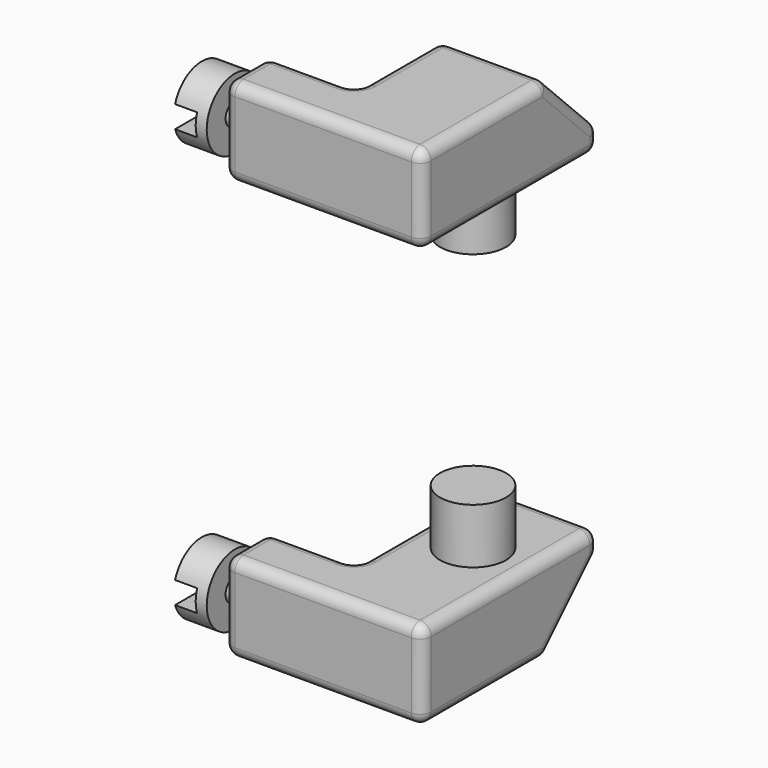
from build123d import *

# Parameters (mm, degrees)
F0_W      = 5
F0_H      = 10
F1_DEPTH  = 4
F2_SIZE   = 3
F3_R      = 1.5
F4_DEPTH  = 2.5
F5_W      = 2.5
F5_H      = 4
F6_DEPTH  = 4
F7_R      = 0.5
F8_R      = 0.5269864315
F9_DEPTH  = 0.5
F10_R     = 1.5960368508
F11_DEPTH = 1.5
F12_W     = 4.0138932984
F12_H     = 1
F13_DEPTH = 1


with BuildPart() as f1:
    # F0 (on Top) → F1 (new body)
    with BuildSketch(Plane.XY):
        Rectangle(F0_W, F0_H)
    extrude(amount=F1_DEPTH)

    # F2
    f2_edges = [f1.edges().sort_by_distance(p)[0] for p in [
        (0, 5, 4),
    ]]
    chamfer(f2_edges, length=F2_SIZE)

    # F3 (on face) → F4 (join)
    with BuildSketch(Plane(origin=(0, 0, 0), x_dir=(1, 0, 0), z_dir=(0, 0, -1))):
        with Locations((0, -1)):
            Circle(F3_R)
    extrude(amount=F4_DEPTH)

    # F5 (on face) → F6 (join)
    with BuildSketch(Plane(origin=(-2.5, 0, 0), x_dir=(0, -1, 0), z_dir=(-1, 0, 0))):
        with Locations((3.75, 2)):
            Rectangle(F5_W, F5_H)
    extrude(amount=F6_DEPTH)

    # F7
    f7_edges = [f1.edges().sort_by_distance(p)[0] for p in [
        (-2.5, -2.5, 2),
        (2.5, -5, 2),
        (0, 5, 0),
        (0, 5, 1),
        (2.5, 3.5, 2.5),
        (0, 2, 4),
        (2.5, 5, 0.5),
        (-2.5, 3.5, 2.5),
        (-2.5, 5, 0.5),
        (-2.5, 1.25, 0),
        (2.5, 0, 0),
        (-2, -5, 0),
        (-2, -5, 4),
        (2.5, -1.5, 4),
        (-2.5, -0.25, 4),
        (-6.5, -5, 2),
        (-6.5, -3.75, 4),
        (-6.5, -2.5, 2),
        (-6.5, -3.75, 0),
        (-4.5, -2.5, 4),
        (-4.5, -2.5, 0),
    ]]
    fillet(f7_edges, radius=F7_R)

    # F8 (on face) → F9 (join)
    with BuildSketch(Plane(origin=(-6.5, 0, 0), x_dir=(0, -1, 0), z_dir=(-1, 0, 0))):
        with Locations((3.75, 2)):
            Circle(F8_R)
    extrude(amount=F9_DEPTH)

    # F10 (on face) → F11 (join)
    with BuildSketch(Plane(origin=(-7, 0, 0), x_dir=(0, -1, 0), z_dir=(-1, 0, 0))):
        with Locations((3.75, 2)):
            Circle(F10_R)
    extrude(amount=F11_DEPTH)

    # F12 (on face) → F13 (cut)
    with BuildSketch(Plane(origin=(-8.5, 0, 0), x_dir=(0, -1, 0), z_dir=(-1, 0, 0))):
        with Locations((3.75, 2)):
            Rectangle(F12_W, F12_H)
    extrude(amount=-F13_DEPTH, mode=Mode.SUBTRACT)


with BuildPart() as f15_1:
    # F15: instance of F1
    add(f1.part.mirror(Plane(origin=(0, 1, -7.5), x_dir=(1, 0, 0), z_dir=(0, 0, -1))))


solid = Compound([f1.part, f15_1.part])
